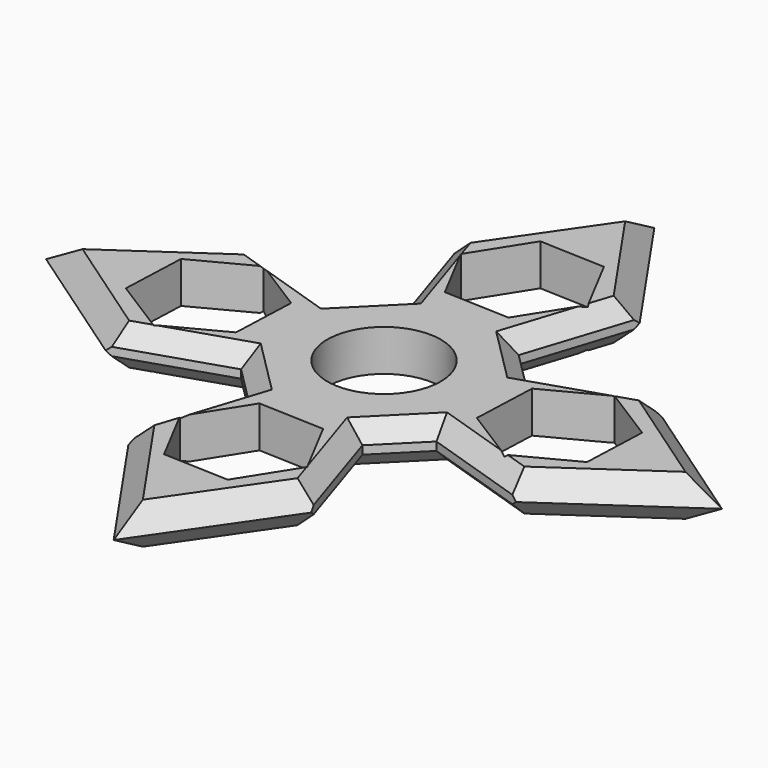
from build123d import *

# Parameters (mm, degrees)
F0_R          = 14.2875
F0_R_2        = 8.7122
F1_DEPTH      = 6.35
F2_T4_DEPTH   = 21.991422614
F2_T10_DEPTH  = 21.991422614
F2_T16_DEPTH  = 30.4110789775
F2_T21_DEPTH  = 30.4110789775
F2_T26_DEPTH  = 30.4110789775
F2_T31_DEPTH  = 30.4110789775
F2_T36_DEPTH  = 30.4110789775
F2_T41_DEPTH  = 30.4110789775
F2_T46_DEPTH  = 21.991422614
F2_T52_DEPTH  = 21.991422614
F2_T58_DEPTH  = 30.4110789775
F2_T63_DEPTH  = 30.4110789775
F2_T68_DEPTH  = 30.4110789775
F2_T73_DEPTH  = 30.4110789775
F2_T78_DEPTH  = 21.991422614
F2_T84_DEPTH  = 21.991422614
F2_T90_DEPTH  = 30.4110789775
F2_T95_DEPTH  = 30.4110789775
F2_T100_DEPTH = 30.4110789775
F2_T105_DEPTH = 30.4110789775
F2_T110_DEPTH = 21.991422614
F2_T116_DEPTH = 21.991422614
F2_T122_DEPTH = 30.4110789775
F2_T127_DEPTH = 30.4110789775
F2_T133_DEPTH = 30.4110789775
F2_T137_DEPTH = 21.991422614
F2_T144_DEPTH = 21.991422614
F2_T148_DEPTH = 30.4110789775
F2_T155_DEPTH = 30.4110789775
F2_T159_DEPTH = 21.991422614
F2_T166_DEPTH = 21.991422614
F2_T170_DEPTH = 30.4110789775
F2_T177_DEPTH = 30.4110789775
F2_T181_DEPTH = 21.991422614
F2_T188_DEPTH = 30.4110789775
F2_T192_DEPTH = 21.991422614
F2_T199_DEPTH = 21.991422614
F2_T203_DEPTH = 30.4110789775
F2_T210_DEPTH = 21.991422614
F2_T214_DEPTH = 30.4110789775
F2_T221_DEPTH = 30.4110789775
F2_T225_DEPTH = 21.991422614
F2_T232_DEPTH = 30.4110789775
F2_T236_DEPTH = 21.991422614
F2_T243_DEPTH = 21.991422614
F2_T247_DEPTH = 30.4110789775
F2_T254_DEPTH = 21.991422614
F2_T258_DEPTH = 30.4110789775
F2_T265_DEPTH = 30.4110789775
F2_T269_DEPTH = 21.991422614
F2_T276_DEPTH = 30.4110789775
F2_T280_DEPTH = 21.991422614
F2_T287_DEPTH = 21.991422614
F2_T291_DEPTH = 30.4110789775
F2_T298_DEPTH = 21.991422614
F2_T302_DEPTH = 30.4110789775
F3_SIZE       = 3.17499


# Not quite as in the source:
# - a fillet or chamfer that OpenCascade refuses, or shapes differently, is made with other operations: its cross-section is extruded or revolved along the edge and cut away or added
# - a fillet or chamfer is up to 0.001 mm smaller than in the source, because OpenCascade refuses the exact size


with BuildPart() as f1:
    # F0 (on Top) → F1 (new body)
    with BuildSketch(Plane.XY):
        Polygon((14.986, 8.6734646993), (8.6734646993, 14.986), (-8.6734646993, 14.986), (-14.986, 8.6734646993), (-14.986, -8.6734646993), (-8.6734646993, -14.986), (8.6734646993, -14.986), (14.986, -8.6734646993), align=None)
        Circle(F0_R, mode=Mode.SUBTRACT)
        Circle(F0_R)
        Circle(F0_R_2, mode=Mode.SUBTRACT)
        Polygon((-14.986, -8.6734646993), (-14.986, 8.6734646993), (-31.4839102423, 14.0339606837), (-41.6801795154, 0), (-31.4839102423, -14.0339606837), align=None)
        Polygon((-35.8485269353, -4.6903220641), (-35.4482015271, 5.3837060107), (-26.5236745918, 10.0740280748), (-17.9994730647, 4.6903220641), (-18.3997984729, -5.3837060107), (-27.3243254082, -10.0740280748), align=None, mode=Mode.SUBTRACT)
        Polygon((14.0339606837, -31.4839102423), (8.6734646993, -14.986), (-8.6734646993, -14.986), (-14.0339606837, -31.4839102423), (0, -41.6801795154), align=None)
        Polygon((4.6903220641, -35.8485269353), (-5.3837060107, -35.4482015271), (-10.0740280748, -26.5236745918), (-4.6903220641, -17.9994730647), (5.3837060107, -18.3997984729), (10.0740280748, -27.3243254082), align=None, mode=Mode.SUBTRACT)
        Polygon((31.4839102423, 14.0339606837), (14.986, 8.6734646993), (14.986, -8.6734646993), (31.4839102423, -14.0339606837), (41.6801795154, 0), align=None)
        Polygon((35.8485269353, 4.6903220641), (35.4482015271, -5.3837060107), (26.5236745918, -10.0740280748), (17.9994730647, -4.6903220641), (18.3997984729, 5.3837060107), (27.3243254082, 10.0740280748), align=None, mode=Mode.SUBTRACT)
        Polygon((-8.6734646993, 14.986), (8.6734646993, 14.986), (14.0339606837, 31.4839102423), (0, 41.6801795154), (-14.0339606837, 31.4839102423), align=None)
        Polygon((5.3837060107, 35.4482015271), (10.0740280748, 26.5236745918), (4.6903220641, 17.9994730647), (-5.3837060107, 18.3997984729), (-10.0740280748, 27.3243254082), (-4.6903220641, 35.8485269353), align=None, mode=Mode.SUBTRACT)
        Polygon((-41.6801795154, 0), (-31.4839102423, 14.0339606837), (-51.8401795154, 0), (-31.4839102423, -14.0339606837), align=None)
        Polygon((0, -51.8401795154), (14.0339606837, -31.4839102423), (0, -41.6801795154), (-14.0339606837, -31.4839102423), align=None)
        Polygon((51.8401795154, 0), (31.4839102423, 14.0339606837), (41.6801795154, 0), (31.4839102423, -14.0339606837), align=None)
        Polygon((0, 41.6801795154), (14.0339606837, 31.4839102423), (0, 51.8401795154), (-14.0339606837, 31.4839102423), align=None)
    extrude(amount=F1_DEPTH)

    # F2: chamfer of 2.54 on 24 edges, made by hand


with BuildPart() as f2_tool2:
    # F2_s3 → F2_t4 (new body)
    with BuildSketch(Plane(origin=(-7.7751420292, -7.7751420292, 0), x_dir=(0, 0, 1), z_dir=(0.7071067812, 0.7071067812, 0))):
        Polygon((3.81, 16.7297679281), (6.35, 14.1897679281), (6.35, 16.7297679281), align=None)
    extrude(amount=F2_T4_DEPTH)

    split(bisect_by=Plane(origin=(3.4409476252, 1.1180316571, 0), x_dir=(0, 0, 1), z_dir=(0.9510565163, 0.3090169944, 0)), keep=Keep.TOP)

    split(bisect_by=Plane(origin=(-1.1180316571, -3.4409476252, 0), x_dir=(0, 0, 1), z_dir=(-0.3090169944, -0.9510565163, 0)), keep=Keep.TOP)


with BuildPart() as f1_1:
    add(f1.part)

    # F2_t1: cut F2_tool2
    add(f2_tool2.part, mode=Mode.SUBTRACT)


with BuildPart() as f2_tool8:
    # F2_s9 → F2_t10 (new body)
    with BuildSketch(Plane(origin=(-7.7751420292, -7.7751420292, 0), x_dir=(0, 0, 1), z_dir=(0.7071067812, 0.7071067812, 0))):
        Polygon((2.54, 16.7297679281), (0, 14.1897679281), (0, 16.7297679281), align=None)
    extrude(amount=F2_T10_DEPTH)

    split(bisect_by=Plane(origin=(3.4409476252, 1.1180316571, 0), x_dir=(0, 0, 1), z_dir=(0.9510565163, 0.3090169944, 0)), keep=Keep.TOP)

    split(bisect_by=Plane(origin=(-1.1180316571, -3.4409476252, 0), x_dir=(0, 0, 1), z_dir=(-0.3090169944, -0.9510565163, 0)), keep=Keep.TOP)


with BuildPart() as f1_2:
    add(f1_1.part)

    # F2_t7: cut F2_tool8
    add(f2_tool8.part, mode=Mode.SUBTRACT)


with BuildPart() as f2_tool14:
    # F2_s15 → F2_t16 (new body)
    with BuildSketch(Plane(origin=(12.611535177, -38.8143141928, 0), x_dir=(0, 0, 1), z_dir=(-0.3090169944, 0.9510565163, 0))):
        Polygon((2.54, 3.6180264434), (0, 1.0780264434), (0, 3.6180264434), align=None)
    extrude(amount=F2_T16_DEPTH)

    split(bisect_by=Plane(origin=(11.8297323497, -11.8297323497, 0), x_dir=(0, 0, 1), z_dir=(0.7071067812, -0.7071067812, 0)), keep=Keep.TOP)


with BuildPart() as f1_3:
    add(f1_2.part)

    # F2_t13: cut F2_tool14
    add(f2_tool14.part, mode=Mode.SUBTRACT)


with BuildPart() as f2_tool19:
    # F2_s20 → F2_t21 (new body)
    with BuildSketch(Plane(origin=(12.611535177, -38.8143141928, 0), x_dir=(0, 0, 1), z_dir=(-0.3090169944, 0.9510565163, 0))):
        Polygon((3.81, 3.6180264434), (6.35, 1.0780264434), (6.35, 3.6180264434), align=None)
    extrude(amount=F2_T21_DEPTH)

    split(bisect_by=Plane(origin=(11.8297323497, -11.8297323497, 0), x_dir=(0, 0, 1), z_dir=(0.7071067812, -0.7071067812, 0)), keep=Keep.TOP)


with BuildPart() as f1_4:
    add(f1_3.part)

    # F2_t18: cut F2_tool19
    add(f2_tool19.part, mode=Mode.SUBTRACT)


with BuildPart() as f2_tool24:
    # F2_s25 → F2_t26 (new body)
    with BuildSketch(Plane(origin=(9.8916593637, -3.2139949557, 0), x_dir=(0, 0, 1), z_dir=(0.9510565163, -0.3090169944, 0))):
        Polygon((2.54, 3.6180264434), (0, 1.0780264434), (0, 3.6180264434), align=None)
    extrude(amount=F2_T26_DEPTH)

    split(bisect_by=Plane(origin=(11.8297323497, -11.8297323497, 0), x_dir=(0, 0, 1), z_dir=(0.7071067812, -0.7071067812, 0)), keep=Keep.TOP)


with BuildPart() as f1_5:
    add(f1_4.part)

    # F2_t23: cut F2_tool24
    add(f2_tool24.part, mode=Mode.SUBTRACT)


with BuildPart() as f2_tool29:
    # F2_s30 → F2_t31 (new body)
    with BuildSketch(Plane(origin=(9.8916593637, -3.2139949557, 0), x_dir=(0, 0, 1), z_dir=(0.9510565163, -0.3090169944, 0))):
        Polygon((3.81, 3.6180264434), (6.35, 1.0780264434), (6.35, 3.6180264434), align=None)
    extrude(amount=F2_T31_DEPTH)

    split(bisect_by=Plane(origin=(11.8297323497, -11.8297323497, 0), x_dir=(0, 0, 1), z_dir=(0.7071067812, -0.7071067812, 0)), keep=Keep.TOP)


with BuildPart() as f1_6:
    add(f1_5.part)

    # F2_t28: cut F2_tool29
    add(f2_tool29.part, mode=Mode.SUBTRACT)


with BuildPart() as f2_tool34:
    # F2_s35 → F2_t36 (new body)
    with BuildSketch(Plane(origin=(38.8143141928, 12.611535177, 0), x_dir=(0, 0, 1), z_dir=(-0.9510565163, -0.3090169944, 0))):
        Polygon((3.81, 3.6180264434), (6.35, 1.0780264434), (6.35, 3.6180264434), align=None)
    extrude(amount=F2_T36_DEPTH)

    split(bisect_by=Plane(origin=(11.8297323497, 11.8297323497, 0), x_dir=(0, 0, 1), z_dir=(0.7071067812, 0.7071067812, 0)), keep=Keep.TOP)


with BuildPart() as f1_7:
    add(f1_6.part)

    # F2_t33: cut F2_tool34
    add(f2_tool34.part, mode=Mode.SUBTRACT)


with BuildPart() as f2_tool39:
    # F2_s40 → F2_t41 (new body)
    with BuildSketch(Plane(origin=(38.8143141928, 12.611535177, 0), x_dir=(0, 0, 1), z_dir=(-0.9510565163, -0.3090169944, 0))):
        Polygon((2.54, 3.6180264434), (0, 1.0780264434), (0, 3.6180264434), align=None)
    extrude(amount=F2_T41_DEPTH)

    split(bisect_by=Plane(origin=(11.8297323497, 11.8297323497, 0), x_dir=(0, 0, 1), z_dir=(0.7071067812, 0.7071067812, 0)), keep=Keep.TOP)


with BuildPart() as f1_8:
    add(f1_7.part)

    # F2_t38: cut F2_tool39
    add(f2_tool39.part, mode=Mode.SUBTRACT)


with BuildPart() as f2_tool44:
    # F2_s45 → F2_t46 (new body)
    with BuildSketch(Plane(origin=(7.7751420292, -7.7751420292, 0), x_dir=(0, 0, 1), z_dir=(-0.7071067812, 0.7071067812, 0))):
        Polygon((2.54, 16.7297679281), (0, 14.1897679281), (0, 16.7297679281), align=None)
    extrude(amount=F2_T46_DEPTH)

    split(bisect_by=Plane(origin=(-1.1180316571, 3.4409476252, 0), x_dir=(0, 0, 1), z_dir=(-0.3090169944, 0.9510565163, 0)), keep=Keep.TOP)

    split(bisect_by=Plane(origin=(3.4409476252, -1.1180316571, 0), x_dir=(0, 0, 1), z_dir=(0.9510565163, -0.3090169944, 0)), keep=Keep.TOP)


with BuildPart() as f1_9:
    add(f1_8.part)

    # F2_t43: cut F2_tool44
    add(f2_tool44.part, mode=Mode.SUBTRACT)


with BuildPart() as f2_tool50:
    # F2_s51 → F2_t52 (new body)
    with BuildSketch(Plane(origin=(7.7751420292, -7.7751420292, 0), x_dir=(0, 0, 1), z_dir=(-0.7071067812, 0.7071067812, 0))):
        Polygon((3.81, 16.7297679281), (6.35, 14.1897679281), (6.35, 16.7297679281), align=None)
    extrude(amount=F2_T52_DEPTH)

    split(bisect_by=Plane(origin=(-1.1180316571, 3.4409476252, 0), x_dir=(0, 0, 1), z_dir=(-0.3090169944, 0.9510565163, 0)), keep=Keep.TOP)

    split(bisect_by=Plane(origin=(3.4409476252, -1.1180316571, 0), x_dir=(0, 0, 1), z_dir=(0.9510565163, -0.3090169944, 0)), keep=Keep.TOP)


with BuildPart() as f1_10:
    add(f1_9.part)

    # F2_t49: cut F2_tool50
    add(f2_tool50.part, mode=Mode.SUBTRACT)


with BuildPart() as f2_tool56:
    # F2_s57 → F2_t58 (new body)
    with BuildSketch(Plane(origin=(3.2139949557, 9.8916593637, 0), x_dir=(0, 0, 1), z_dir=(0.3090169944, 0.9510565163, 0))):
        Polygon((2.54, 3.6180264434), (0, 1.0780264434), (0, 3.6180264434), align=None)
    extrude(amount=F2_T58_DEPTH)

    split(bisect_by=Plane(origin=(11.8297323497, 11.8297323497, 0), x_dir=(0, 0, 1), z_dir=(0.7071067812, 0.7071067812, 0)), keep=Keep.TOP)


with BuildPart() as f1_11:
    add(f1_10.part)

    # F2_t55: cut F2_tool56
    add(f2_tool56.part, mode=Mode.SUBTRACT)


with BuildPart() as f2_tool61:
    # F2_s62 → F2_t63 (new body)
    with BuildSketch(Plane(origin=(3.2139949557, 9.8916593637, 0), x_dir=(0, 0, 1), z_dir=(0.3090169944, 0.9510565163, 0))):
        Polygon((3.81, 3.6180264434), (6.35, 1.0780264434), (6.35, 3.6180264434), align=None)
    extrude(amount=F2_T63_DEPTH)

    split(bisect_by=Plane(origin=(11.8297323497, 11.8297323497, 0), x_dir=(0, 0, 1), z_dir=(0.7071067812, 0.7071067812, 0)), keep=Keep.TOP)


with BuildPart() as f1_12:
    add(f1_11.part)

    # F2_t60: cut F2_tool61
    add(f2_tool61.part, mode=Mode.SUBTRACT)


with BuildPart() as f2_tool66:
    # F2_s67 → F2_t68 (new body)
    with BuildSketch(Plane(origin=(-12.611535177, 38.8143141928, 0), x_dir=(0, 0, 1), z_dir=(0.3090169944, -0.9510565163, 0))):
        Polygon((3.81, 3.6180264434), (6.35, 1.0780264434), (6.35, 3.6180264434), align=None)
    extrude(amount=F2_T68_DEPTH)

    split(bisect_by=Plane(origin=(-11.8297323497, 11.8297323497, 0), x_dir=(0, 0, 1), z_dir=(-0.7071067812, 0.7071067812, 0)), keep=Keep.TOP)


with BuildPart() as f1_13:
    add(f1_12.part)

    # F2_t65: cut F2_tool66
    add(f2_tool66.part, mode=Mode.SUBTRACT)


with BuildPart() as f2_tool71:
    # F2_s72 → F2_t73 (new body)
    with BuildSketch(Plane(origin=(-12.611535177, 38.8143141928, 0), x_dir=(0, 0, 1), z_dir=(0.3090169944, -0.9510565163, 0))):
        Polygon((2.54, 3.6180264434), (0, 1.0780264434), (0, 3.6180264434), align=None)
    extrude(amount=F2_T73_DEPTH)

    split(bisect_by=Plane(origin=(-11.8297323497, 11.8297323497, 0), x_dir=(0, 0, 1), z_dir=(-0.7071067812, 0.7071067812, 0)), keep=Keep.TOP)


with BuildPart() as f1_14:
    add(f1_13.part)

    # F2_t70: cut F2_tool71
    add(f2_tool71.part, mode=Mode.SUBTRACT)


with BuildPart() as f2_tool76:
    # F2_s77 → F2_t78 (new body)
    with BuildSketch(Plane(origin=(7.7751420292, 7.7751420292, 0), x_dir=(0, 0, 1), z_dir=(-0.7071067812, -0.7071067812, 0))):
        Polygon((3.81, 16.7297679281), (6.35, 14.1897679281), (6.35, 16.7297679281), align=None)
    extrude(amount=F2_T78_DEPTH)

    split(bisect_by=Plane(origin=(-3.4409476252, -1.1180316571, 0), x_dir=(0, 0, 1), z_dir=(-0.9510565163, -0.3090169944, 0)), keep=Keep.TOP)

    split(bisect_by=Plane(origin=(1.1180316571, 3.4409476252, 0), x_dir=(0, 0, 1), z_dir=(0.3090169944, 0.9510565163, 0)), keep=Keep.TOP)


with BuildPart() as f1_15:
    add(f1_14.part)

    # F2_t75: cut F2_tool76
    add(f2_tool76.part, mode=Mode.SUBTRACT)


with BuildPart() as f2_tool82:
    # F2_s83 → F2_t84 (new body)
    with BuildSketch(Plane(origin=(7.7751420292, 7.7751420292, 0), x_dir=(0, 0, 1), z_dir=(-0.7071067812, -0.7071067812, 0))):
        Polygon((2.54, 16.7297679281), (0, 14.1897679281), (0, 16.7297679281), align=None)
    extrude(amount=F2_T84_DEPTH)

    split(bisect_by=Plane(origin=(-3.4409476252, -1.1180316571, 0), x_dir=(0, 0, 1), z_dir=(-0.9510565163, -0.3090169944, 0)), keep=Keep.TOP)

    split(bisect_by=Plane(origin=(1.1180316571, 3.4409476252, 0), x_dir=(0, 0, 1), z_dir=(0.3090169944, 0.9510565163, 0)), keep=Keep.TOP)


with BuildPart() as f1_16:
    add(f1_15.part)

    # F2_t81: cut F2_tool82
    add(f2_tool82.part, mode=Mode.SUBTRACT)


with BuildPart() as f2_tool88:
    # F2_s89 → F2_t90 (new body)
    with BuildSketch(Plane(origin=(-9.8916593637, 3.2139949557, 0), x_dir=(0, 0, 1), z_dir=(-0.9510565163, 0.3090169944, 0))):
        Polygon((2.54, 3.6180264434), (0, 1.0780264434), (0, 3.6180264434), align=None)
    extrude(amount=F2_T90_DEPTH)

    split(bisect_by=Plane(origin=(-11.8297323497, 11.8297323497, 0), x_dir=(0, 0, 1), z_dir=(-0.7071067812, 0.7071067812, 0)), keep=Keep.TOP)


with BuildPart() as f1_17:
    add(f1_16.part)

    # F2_t87: cut F2_tool88
    add(f2_tool88.part, mode=Mode.SUBTRACT)


with BuildPart() as f2_tool93:
    # F2_s94 → F2_t95 (new body)
    with BuildSketch(Plane(origin=(-9.8916593637, 3.2139949557, 0), x_dir=(0, 0, 1), z_dir=(-0.9510565163, 0.3090169944, 0))):
        Polygon((3.81, 3.6180264434), (6.35, 1.0780264434), (6.35, 3.6180264434), align=None)
    extrude(amount=F2_T95_DEPTH)

    split(bisect_by=Plane(origin=(-11.8297323497, 11.8297323497, 0), x_dir=(0, 0, 1), z_dir=(-0.7071067812, 0.7071067812, 0)), keep=Keep.TOP)


with BuildPart() as f1_18:
    add(f1_17.part)

    # F2_t92: cut F2_tool93
    add(f2_tool93.part, mode=Mode.SUBTRACT)


with BuildPart() as f2_tool98:
    # F2_s99 → F2_t100 (new body)
    with BuildSketch(Plane(origin=(-38.8143141928, -12.611535177, 0), x_dir=(0, 0, 1), z_dir=(0.9510565163, 0.3090169944, 0))):
        Polygon((3.81, 3.6180264434), (6.35, 1.0780264434), (6.35, 3.6180264434), align=None)
    extrude(amount=F2_T100_DEPTH)

    split(bisect_by=Plane(origin=(-11.8297323497, -11.8297323497, 0), x_dir=(0, 0, 1), z_dir=(-0.7071067812, -0.7071067812, 0)), keep=Keep.TOP)


with BuildPart() as f1_19:
    add(f1_18.part)

    # F2_t97: cut F2_tool98
    add(f2_tool98.part, mode=Mode.SUBTRACT)


with BuildPart() as f2_tool103:
    # F2_s104 → F2_t105 (new body)
    with BuildSketch(Plane(origin=(-38.8143141928, -12.611535177, 0), x_dir=(0, 0, 1), z_dir=(0.9510565163, 0.3090169944, 0))):
        Polygon((2.54, 3.6180264434), (0, 1.0780264434), (0, 3.6180264434), align=None)
    extrude(amount=F2_T105_DEPTH)

    split(bisect_by=Plane(origin=(-11.8297323497, -11.8297323497, 0), x_dir=(0, 0, 1), z_dir=(-0.7071067812, -0.7071067812, 0)), keep=Keep.TOP)


with BuildPart() as f1_20:
    add(f1_19.part)

    # F2_t102: cut F2_tool103
    add(f2_tool103.part, mode=Mode.SUBTRACT)


with BuildPart() as f2_tool108:
    # F2_s109 → F2_t110 (new body)
    with BuildSketch(Plane(origin=(-7.7751420292, 7.7751420292, 0), x_dir=(0, 0, 1), z_dir=(0.7071067812, -0.7071067812, 0))):
        Polygon((3.81, 16.7297679281), (6.35, 14.1897679281), (6.35, 16.7297679281), align=None)
    extrude(amount=F2_T110_DEPTH)

    split(bisect_by=Plane(origin=(1.1180316571, -3.4409476252, 0), x_dir=(0, 0, 1), z_dir=(0.3090169944, -0.9510565163, 0)), keep=Keep.TOP)

    split(bisect_by=Plane(origin=(-3.4409476252, 1.1180316571, 0), x_dir=(0, 0, 1), z_dir=(-0.9510565163, 0.3090169944, 0)), keep=Keep.TOP)


with BuildPart() as f1_21:
    add(f1_20.part)

    # F2_t107: cut F2_tool108
    add(f2_tool108.part, mode=Mode.SUBTRACT)


with BuildPart() as f2_tool114:
    # F2_s115 → F2_t116 (new body)
    with BuildSketch(Plane(origin=(-7.7751420292, 7.7751420292, 0), x_dir=(0, 0, 1), z_dir=(0.7071067812, -0.7071067812, 0))):
        Polygon((2.54, 16.7297679281), (0, 14.1897679281), (0, 16.7297679281), align=None)
    extrude(amount=F2_T116_DEPTH)

    split(bisect_by=Plane(origin=(1.1180316571, -3.4409476252, 0), x_dir=(0, 0, 1), z_dir=(0.3090169944, -0.9510565163, 0)), keep=Keep.TOP)

    split(bisect_by=Plane(origin=(-3.4409476252, 1.1180316571, 0), x_dir=(0, 0, 1), z_dir=(-0.9510565163, 0.3090169944, 0)), keep=Keep.TOP)


with BuildPart() as f1_22:
    add(f1_21.part)

    # F2_t113: cut F2_tool114
    add(f2_tool114.part, mode=Mode.SUBTRACT)


with BuildPart() as f2_tool120:
    # F2_s121 → F2_t122 (new body)
    with BuildSketch(Plane(origin=(-3.2139949557, -9.8916593637, 0), x_dir=(0, 0, 1), z_dir=(-0.3090169944, -0.9510565163, 0))):
        Polygon((3.81, 3.6180264434), (6.35, 1.0780264434), (6.35, 3.6180264434), align=None)
    extrude(amount=F2_T122_DEPTH)

    split(bisect_by=Plane(origin=(-11.8297323497, -11.8297323497, 0), x_dir=(0, 0, 1), z_dir=(-0.7071067812, -0.7071067812, 0)), keep=Keep.TOP)


with BuildPart() as f1_23:
    add(f1_22.part)

    # F2_t119: cut F2_tool120
    add(f2_tool120.part, mode=Mode.SUBTRACT)


with BuildPart() as f2_tool125:
    # F2_s126 → F2_t127 (new body)
    with BuildSketch(Plane(origin=(-3.2139949557, -9.8916593637, 0), x_dir=(0, 0, 1), z_dir=(-0.3090169944, -0.9510565163, 0))):
        Polygon((2.54, 3.6180264434), (0, 1.0780264434), (0, 3.6180264434), align=None)
    extrude(amount=F2_T127_DEPTH)

    split(bisect_by=Plane(origin=(-11.8297323497, -11.8297323497, 0), x_dir=(0, 0, 1), z_dir=(-0.7071067812, -0.7071067812, 0)), keep=Keep.TOP)


with BuildPart() as f1_24:
    add(f1_23.part)

    # F2_t124: cut F2_tool125
    add(f2_tool125.part, mode=Mode.SUBTRACT)


with BuildPart() as f2_tool131:
    # F2_s132 → F2_t133 (new body)
    with BuildSketch(Plane(origin=(12.611535177, -38.8143141928, 0), x_dir=(0, 0, 1), z_dir=(-0.3090169944, 0.9510565163, 0))):
        Polygon((3.81, 3.6180264434), (6.35, 1.0780264434), (6.35, 3.6180264434), align=None)
    extrude(amount=F2_T133_DEPTH)

    split(bisect_by=Plane(origin=(11.8297323497, -11.8297323497, 0), x_dir=(0, 0, 1), z_dir=(-0.7071067812, 0.7071067812, 0)), keep=Keep.TOP)


with BuildPart() as f2_tool135:
    # F2_s136 → F2_t137 (new body)
    with BuildSketch(Plane(origin=(-7.7751420292, -7.7751420292, 0), x_dir=(0, 0, 1), z_dir=(0.7071067812, 0.7071067812, 0))):
        Polygon((3.81, 16.7297679281), (6.35, 14.1897679281), (6.35, 16.7297679281), align=None)
    extrude(amount=F2_T137_DEPTH)

    split(bisect_by=Plane(origin=(3.4409476252, 1.1180316571, 0), x_dir=(0, 0, 1), z_dir=(-0.9510565163, -0.3090169944, 0)), keep=Keep.TOP)


with BuildPart() as f2_tool131_1:
    add(f2_tool131.part)

    # F2_t139: intersect F2_tool135
    add(f2_tool135.part, mode=Mode.INTERSECT)


with BuildPart() as f1_25:
    add(f1_24.part)

    # F2_t129: cut F2_tool131
    add(f2_tool131_1.part, mode=Mode.SUBTRACT)


with BuildPart() as f2_tool142:
    # F2_s143 → F2_t144 (new body)
    with BuildSketch(Plane(origin=(-7.7751420292, -7.7751420292, 0), x_dir=(0, 0, 1), z_dir=(0.7071067812, 0.7071067812, 0))):
        Polygon((3.81, 16.7297679281), (6.35, 14.1897679281), (6.35, 16.7297679281), align=None)
    extrude(amount=F2_T144_DEPTH)

    split(bisect_by=Plane(origin=(-1.1180316571, -3.4409476252, 0), x_dir=(0, 0, 1), z_dir=(0.3090169944, 0.9510565163, 0)), keep=Keep.TOP)


with BuildPart() as f2_tool146:
    # F2_s147 → F2_t148 (new body)
    with BuildSketch(Plane(origin=(9.8916593637, -3.2139949557, 0), x_dir=(0, 0, 1), z_dir=(0.9510565163, -0.3090169944, 0))):
        Polygon((3.81, 3.6180264434), (6.35, 1.0780264434), (6.35, 3.6180264434), align=None)
    extrude(amount=F2_T148_DEPTH)

    split(bisect_by=Plane(origin=(11.8297323497, -11.8297323497, 0), x_dir=(0, 0, 1), z_dir=(-0.7071067812, 0.7071067812, 0)), keep=Keep.TOP)


with BuildPart() as f2_tool142_1:
    add(f2_tool142.part)

    # F2_t150: intersect F2_tool146
    add(f2_tool146.part, mode=Mode.INTERSECT)


with BuildPart() as f1_26:
    add(f1_25.part)

    # F2_t140: cut F2_tool142
    add(f2_tool142_1.part, mode=Mode.SUBTRACT)


with BuildPart() as f2_tool153:
    # F2_s154 → F2_t155 (new body)
    with BuildSketch(Plane(origin=(12.611535177, -38.8143141928, 0), x_dir=(0, 0, 1), z_dir=(-0.3090169944, 0.9510565163, 0))):
        Polygon((2.54, 3.6180264434), (0, 1.0780264434), (0, 3.6180264434), align=None)
    extrude(amount=F2_T155_DEPTH)

    split(bisect_by=Plane(origin=(11.8297323497, -11.8297323497, 0), x_dir=(0, 0, 1), z_dir=(-0.7071067812, 0.7071067812, 0)), keep=Keep.TOP)


with BuildPart() as f2_tool157:
    # F2_s158 → F2_t159 (new body)
    with BuildSketch(Plane(origin=(-7.7751420292, -7.7751420292, 0), x_dir=(0, 0, 1), z_dir=(0.7071067812, 0.7071067812, 0))):
        Polygon((2.54, 16.7297679281), (0, 14.1897679281), (0, 16.7297679281), align=None)
    extrude(amount=F2_T159_DEPTH)

    split(bisect_by=Plane(origin=(3.4409476252, 1.1180316571, 0), x_dir=(0, 0, 1), z_dir=(-0.9510565163, -0.3090169944, 0)), keep=Keep.TOP)


with BuildPart() as f2_tool153_1:
    add(f2_tool153.part)

    # F2_t161: intersect F2_tool157
    add(f2_tool157.part, mode=Mode.INTERSECT)


with BuildPart() as f1_27:
    add(f1_26.part)

    # F2_t151: cut F2_tool153
    add(f2_tool153_1.part, mode=Mode.SUBTRACT)


with BuildPart() as f2_tool164:
    # F2_s165 → F2_t166 (new body)
    with BuildSketch(Plane(origin=(-7.7751420292, -7.7751420292, 0), x_dir=(0, 0, 1), z_dir=(0.7071067812, 0.7071067812, 0))):
        Polygon((2.54, 16.7297679281), (0, 14.1897679281), (0, 16.7297679281), align=None)
    extrude(amount=F2_T166_DEPTH)

    split(bisect_by=Plane(origin=(-1.1180316571, -3.4409476252, 0), x_dir=(0, 0, 1), z_dir=(0.3090169944, 0.9510565163, 0)), keep=Keep.TOP)


with BuildPart() as f2_tool168:
    # F2_s169 → F2_t170 (new body)
    with BuildSketch(Plane(origin=(9.8916593637, -3.2139949557, 0), x_dir=(0, 0, 1), z_dir=(0.9510565163, -0.3090169944, 0))):
        Polygon((2.54, 3.6180264434), (0, 1.0780264434), (0, 3.6180264434), align=None)
    extrude(amount=F2_T170_DEPTH)

    split(bisect_by=Plane(origin=(11.8297323497, -11.8297323497, 0), x_dir=(0, 0, 1), z_dir=(-0.7071067812, 0.7071067812, 0)), keep=Keep.TOP)


with BuildPart() as f2_tool164_1:
    add(f2_tool164.part)

    # F2_t172: intersect F2_tool168
    add(f2_tool168.part, mode=Mode.INTERSECT)


with BuildPart() as f1_28:
    add(f1_27.part)

    # F2_t162: cut F2_tool164
    add(f2_tool164_1.part, mode=Mode.SUBTRACT)


with BuildPart() as f2_tool175:
    # F2_s176 → F2_t177 (new body)
    with BuildSketch(Plane(origin=(38.8143141928, 12.611535177, 0), x_dir=(0, 0, 1), z_dir=(-0.9510565163, -0.3090169944, 0))):
        Polygon((3.81, 3.6180264434), (6.35, 1.0780264434), (6.35, 3.6180264434), align=None)
    extrude(amount=F2_T177_DEPTH)

    split(bisect_by=Plane(origin=(11.8297323497, 11.8297323497, 0), x_dir=(0, 0, 1), z_dir=(-0.7071067812, -0.7071067812, 0)), keep=Keep.TOP)


with BuildPart() as f2_tool179:
    # F2_s180 → F2_t181 (new body)
    with BuildSketch(Plane(origin=(7.7751420292, -7.7751420292, 0), x_dir=(0, 0, 1), z_dir=(-0.7071067812, 0.7071067812, 0))):
        Polygon((3.81, 16.7297679281), (6.35, 14.1897679281), (6.35, 16.7297679281), align=None)
    extrude(amount=F2_T181_DEPTH)

    split(bisect_by=Plane(origin=(-1.1180316571, 3.4409476252, 0), x_dir=(0, 0, 1), z_dir=(0.3090169944, -0.9510565163, 0)), keep=Keep.TOP)


with BuildPart() as f2_tool175_1:
    add(f2_tool175.part)

    # F2_t183: intersect F2_tool179
    add(f2_tool179.part, mode=Mode.INTERSECT)


with BuildPart() as f1_29:
    add(f1_28.part)

    # F2_t173: cut F2_tool175
    add(f2_tool175_1.part, mode=Mode.SUBTRACT)


with BuildPart() as f2_tool186:
    # F2_s187 → F2_t188 (new body)
    with BuildSketch(Plane(origin=(38.8143141928, 12.611535177, 0), x_dir=(0, 0, 1), z_dir=(-0.9510565163, -0.3090169944, 0))):
        Polygon((2.54, 3.6180264434), (0, 1.0780264434), (0, 3.6180264434), align=None)
    extrude(amount=F2_T188_DEPTH)

    split(bisect_by=Plane(origin=(11.8297323497, 11.8297323497, 0), x_dir=(0, 0, 1), z_dir=(-0.7071067812, -0.7071067812, 0)), keep=Keep.TOP)


with BuildPart() as f2_tool190:
    # F2_s191 → F2_t192 (new body)
    with BuildSketch(Plane(origin=(7.7751420292, -7.7751420292, 0), x_dir=(0, 0, 1), z_dir=(-0.7071067812, 0.7071067812, 0))):
        Polygon((2.54, 16.7297679281), (0, 14.1897679281), (0, 16.7297679281), align=None)
    extrude(amount=F2_T192_DEPTH)

    split(bisect_by=Plane(origin=(-1.1180316571, 3.4409476252, 0), x_dir=(0, 0, 1), z_dir=(0.3090169944, -0.9510565163, 0)), keep=Keep.TOP)


with BuildPart() as f2_tool186_1:
    add(f2_tool186.part)

    # F2_t194: intersect F2_tool190
    add(f2_tool190.part, mode=Mode.INTERSECT)


with BuildPart() as f1_30:
    add(f1_29.part)

    # F2_t184: cut F2_tool186
    add(f2_tool186_1.part, mode=Mode.SUBTRACT)


with BuildPart() as f2_tool197:
    # F2_s198 → F2_t199 (new body)
    with BuildSketch(Plane(origin=(7.7751420292, -7.7751420292, 0), x_dir=(0, 0, 1), z_dir=(-0.7071067812, 0.7071067812, 0))):
        Polygon((2.54, 16.7297679281), (0, 14.1897679281), (0, 16.7297679281), align=None)
    extrude(amount=F2_T199_DEPTH)

    split(bisect_by=Plane(origin=(3.4409476252, -1.1180316571, 0), x_dir=(0, 0, 1), z_dir=(-0.9510565163, 0.3090169944, 0)), keep=Keep.TOP)


with BuildPart() as f2_tool201:
    # F2_s202 → F2_t203 (new body)
    with BuildSketch(Plane(origin=(3.2139949557, 9.8916593637, 0), x_dir=(0, 0, 1), z_dir=(0.3090169944, 0.9510565163, 0))):
        Polygon((2.54, 3.6180264434), (0, 1.0780264434), (0, 3.6180264434), align=None)
    extrude(amount=F2_T203_DEPTH)

    split(bisect_by=Plane(origin=(11.8297323497, 11.8297323497, 0), x_dir=(0, 0, 1), z_dir=(-0.7071067812, -0.7071067812, 0)), keep=Keep.TOP)


with BuildPart() as f2_tool197_1:
    add(f2_tool197.part)

    # F2_t205: intersect F2_tool201
    add(f2_tool201.part, mode=Mode.INTERSECT)


with BuildPart() as f1_31:
    add(f1_30.part)

    # F2_t195: cut F2_tool197
    add(f2_tool197_1.part, mode=Mode.SUBTRACT)


with BuildPart() as f2_tool208:
    # F2_s209 → F2_t210 (new body)
    with BuildSketch(Plane(origin=(7.7751420292, -7.7751420292, 0), x_dir=(0, 0, 1), z_dir=(-0.7071067812, 0.7071067812, 0))):
        Polygon((3.81, 16.7297679281), (6.35, 14.1897679281), (6.35, 16.7297679281), align=None)
    extrude(amount=F2_T210_DEPTH)

    split(bisect_by=Plane(origin=(3.4409476252, -1.1180316571, 0), x_dir=(0, 0, 1), z_dir=(-0.9510565163, 0.3090169944, 0)), keep=Keep.TOP)


with BuildPart() as f2_tool212:
    # F2_s213 → F2_t214 (new body)
    with BuildSketch(Plane(origin=(3.2139949557, 9.8916593637, 0), x_dir=(0, 0, 1), z_dir=(0.3090169944, 0.9510565163, 0))):
        Polygon((3.81, 3.6180264434), (6.35, 1.0780264434), (6.35, 3.6180264434), align=None)
    extrude(amount=F2_T214_DEPTH)

    split(bisect_by=Plane(origin=(11.8297323497, 11.8297323497, 0), x_dir=(0, 0, 1), z_dir=(-0.7071067812, -0.7071067812, 0)), keep=Keep.TOP)


with BuildPart() as f2_tool208_1:
    add(f2_tool208.part)

    # F2_t216: intersect F2_tool212
    add(f2_tool212.part, mode=Mode.INTERSECT)


with BuildPart() as f1_32:
    add(f1_31.part)

    # F2_t206: cut F2_tool208
    add(f2_tool208_1.part, mode=Mode.SUBTRACT)


with BuildPart() as f2_tool219:
    # F2_s220 → F2_t221 (new body)
    with BuildSketch(Plane(origin=(-12.611535177, 38.8143141928, 0), x_dir=(0, 0, 1), z_dir=(0.3090169944, -0.9510565163, 0))):
        Polygon((3.81, 3.6180264434), (6.35, 1.0780264434), (6.35, 3.6180264434), align=None)
    extrude(amount=F2_T221_DEPTH)

    split(bisect_by=Plane(origin=(-11.8297323497, 11.8297323497, 0), x_dir=(0, 0, 1), z_dir=(0.7071067812, -0.7071067812, 0)), keep=Keep.TOP)


with BuildPart() as f2_tool223:
    # F2_s224 → F2_t225 (new body)
    with BuildSketch(Plane(origin=(7.7751420292, 7.7751420292, 0), x_dir=(0, 0, 1), z_dir=(-0.7071067812, -0.7071067812, 0))):
        Polygon((3.81, 16.7297679281), (6.35, 14.1897679281), (6.35, 16.7297679281), align=None)
    extrude(amount=F2_T225_DEPTH)

    split(bisect_by=Plane(origin=(-3.4409476252, -1.1180316571, 0), x_dir=(0, 0, 1), z_dir=(0.9510565163, 0.3090169944, 0)), keep=Keep.TOP)


with BuildPart() as f2_tool219_1:
    add(f2_tool219.part)

    # F2_t227: intersect F2_tool223
    add(f2_tool223.part, mode=Mode.INTERSECT)


with BuildPart() as f1_33:
    add(f1_32.part)

    # F2_t217: cut F2_tool219
    add(f2_tool219_1.part, mode=Mode.SUBTRACT)


with BuildPart() as f2_tool230:
    # F2_s231 → F2_t232 (new body)
    with BuildSketch(Plane(origin=(-12.611535177, 38.8143141928, 0), x_dir=(0, 0, 1), z_dir=(0.3090169944, -0.9510565163, 0))):
        Polygon((2.54, 3.6180264434), (0, 1.0780264434), (0, 3.6180264434), align=None)
    extrude(amount=F2_T232_DEPTH)

    split(bisect_by=Plane(origin=(-11.8297323497, 11.8297323497, 0), x_dir=(0, 0, 1), z_dir=(0.7071067812, -0.7071067812, 0)), keep=Keep.TOP)


with BuildPart() as f2_tool234:
    # F2_s235 → F2_t236 (new body)
    with BuildSketch(Plane(origin=(7.7751420292, 7.7751420292, 0), x_dir=(0, 0, 1), z_dir=(-0.7071067812, -0.7071067812, 0))):
        Polygon((2.54, 16.7297679281), (0, 14.1897679281), (0, 16.7297679281), align=None)
    extrude(amount=F2_T236_DEPTH)

    split(bisect_by=Plane(origin=(-3.4409476252, -1.1180316571, 0), x_dir=(0, 0, 1), z_dir=(0.9510565163, 0.3090169944, 0)), keep=Keep.TOP)


with BuildPart() as f2_tool230_1:
    add(f2_tool230.part)

    # F2_t238: intersect F2_tool234
    add(f2_tool234.part, mode=Mode.INTERSECT)


with BuildPart() as f1_34:
    add(f1_33.part)

    # F2_t228: cut F2_tool230
    add(f2_tool230_1.part, mode=Mode.SUBTRACT)


with BuildPart() as f2_tool241:
    # F2_s242 → F2_t243 (new body)
    with BuildSketch(Plane(origin=(7.7751420292, 7.7751420292, 0), x_dir=(0, 0, 1), z_dir=(-0.7071067812, -0.7071067812, 0))):
        Polygon((3.81, 16.7297679281), (6.35, 14.1897679281), (6.35, 16.7297679281), align=None)
    extrude(amount=F2_T243_DEPTH)

    split(bisect_by=Plane(origin=(1.1180316571, 3.4409476252, 0), x_dir=(0, 0, 1), z_dir=(-0.3090169944, -0.9510565163, 0)), keep=Keep.TOP)


with BuildPart() as f2_tool245:
    # F2_s246 → F2_t247 (new body)
    with BuildSketch(Plane(origin=(-9.8916593637, 3.2139949557, 0), x_dir=(0, 0, 1), z_dir=(-0.9510565163, 0.3090169944, 0))):
        Polygon((3.81, 3.6180264434), (6.35, 1.0780264434), (6.35, 3.6180264434), align=None)
    extrude(amount=F2_T247_DEPTH)

    split(bisect_by=Plane(origin=(-11.8297323497, 11.8297323497, 0), x_dir=(0, 0, 1), z_dir=(0.7071067812, -0.7071067812, 0)), keep=Keep.TOP)


with BuildPart() as f2_tool241_1:
    add(f2_tool241.part)

    # F2_t249: intersect F2_tool245
    add(f2_tool245.part, mode=Mode.INTERSECT)


with BuildPart() as f1_35:
    add(f1_34.part)

    # F2_t239: cut F2_tool241
    add(f2_tool241_1.part, mode=Mode.SUBTRACT)


with BuildPart() as f2_tool252:
    # F2_s253 → F2_t254 (new body)
    with BuildSketch(Plane(origin=(7.7751420292, 7.7751420292, 0), x_dir=(0, 0, 1), z_dir=(-0.7071067812, -0.7071067812, 0))):
        Polygon((2.54, 16.7297679281), (0, 14.1897679281), (0, 16.7297679281), align=None)
    extrude(amount=F2_T254_DEPTH)

    split(bisect_by=Plane(origin=(1.1180316571, 3.4409476252, 0), x_dir=(0, 0, 1), z_dir=(-0.3090169944, -0.9510565163, 0)), keep=Keep.TOP)


with BuildPart() as f2_tool256:
    # F2_s257 → F2_t258 (new body)
    with BuildSketch(Plane(origin=(-9.8916593637, 3.2139949557, 0), x_dir=(0, 0, 1), z_dir=(-0.9510565163, 0.3090169944, 0))):
        Polygon((2.54, 3.6180264434), (0, 1.0780264434), (0, 3.6180264434), align=None)
    extrude(amount=F2_T258_DEPTH)

    split(bisect_by=Plane(origin=(-11.8297323497, 11.8297323497, 0), x_dir=(0, 0, 1), z_dir=(0.7071067812, -0.7071067812, 0)), keep=Keep.TOP)


with BuildPart() as f2_tool252_1:
    add(f2_tool252.part)

    # F2_t260: intersect F2_tool256
    add(f2_tool256.part, mode=Mode.INTERSECT)


with BuildPart() as f1_36:
    add(f1_35.part)

    # F2_t250: cut F2_tool252
    add(f2_tool252_1.part, mode=Mode.SUBTRACT)


with BuildPart() as f2_tool263:
    # F2_s264 → F2_t265 (new body)
    with BuildSketch(Plane(origin=(-38.8143141928, -12.611535177, 0), x_dir=(0, 0, 1), z_dir=(0.9510565163, 0.3090169944, 0))):
        Polygon((3.81, 3.6180264434), (6.35, 1.0780264434), (6.35, 3.6180264434), align=None)
    extrude(amount=F2_T265_DEPTH)

    split(bisect_by=Plane(origin=(-11.8297323497, -11.8297323497, 0), x_dir=(0, 0, 1), z_dir=(0.7071067812, 0.7071067812, 0)), keep=Keep.TOP)


with BuildPart() as f2_tool267:
    # F2_s268 → F2_t269 (new body)
    with BuildSketch(Plane(origin=(-7.7751420292, 7.7751420292, 0), x_dir=(0, 0, 1), z_dir=(0.7071067812, -0.7071067812, 0))):
        Polygon((3.81, 16.7297679281), (6.35, 14.1897679281), (6.35, 16.7297679281), align=None)
    extrude(amount=F2_T269_DEPTH)

    split(bisect_by=Plane(origin=(1.1180316571, -3.4409476252, 0), x_dir=(0, 0, 1), z_dir=(-0.3090169944, 0.9510565163, 0)), keep=Keep.TOP)


with BuildPart() as f2_tool263_1:
    add(f2_tool263.part)

    # F2_t271: intersect F2_tool267
    add(f2_tool267.part, mode=Mode.INTERSECT)


with BuildPart() as f1_37:
    add(f1_36.part)

    # F2_t261: cut F2_tool263
    add(f2_tool263_1.part, mode=Mode.SUBTRACT)


with BuildPart() as f2_tool274:
    # F2_s275 → F2_t276 (new body)
    with BuildSketch(Plane(origin=(-38.8143141928, -12.611535177, 0), x_dir=(0, 0, 1), z_dir=(0.9510565163, 0.3090169944, 0))):
        Polygon((2.54, 3.6180264434), (0, 1.0780264434), (0, 3.6180264434), align=None)
    extrude(amount=F2_T276_DEPTH)

    split(bisect_by=Plane(origin=(-11.8297323497, -11.8297323497, 0), x_dir=(0, 0, 1), z_dir=(0.7071067812, 0.7071067812, 0)), keep=Keep.TOP)


with BuildPart() as f2_tool278:
    # F2_s279 → F2_t280 (new body)
    with BuildSketch(Plane(origin=(-7.7751420292, 7.7751420292, 0), x_dir=(0, 0, 1), z_dir=(0.7071067812, -0.7071067812, 0))):
        Polygon((2.54, 16.7297679281), (0, 14.1897679281), (0, 16.7297679281), align=None)
    extrude(amount=F2_T280_DEPTH)

    split(bisect_by=Plane(origin=(1.1180316571, -3.4409476252, 0), x_dir=(0, 0, 1), z_dir=(-0.3090169944, 0.9510565163, 0)), keep=Keep.TOP)


with BuildPart() as f2_tool274_1:
    add(f2_tool274.part)

    # F2_t282: intersect F2_tool278
    add(f2_tool278.part, mode=Mode.INTERSECT)


with BuildPart() as f1_38:
    add(f1_37.part)

    # F2_t272: cut F2_tool274
    add(f2_tool274_1.part, mode=Mode.SUBTRACT)


with BuildPart() as f2_tool285:
    # F2_s286 → F2_t287 (new body)
    with BuildSketch(Plane(origin=(-7.7751420292, 7.7751420292, 0), x_dir=(0, 0, 1), z_dir=(0.7071067812, -0.7071067812, 0))):
        Polygon((3.81, 16.7297679281), (6.35, 14.1897679281), (6.35, 16.7297679281), align=None)
    extrude(amount=F2_T287_DEPTH)

    split(bisect_by=Plane(origin=(-3.4409476252, 1.1180316571, 0), x_dir=(0, 0, 1), z_dir=(0.9510565163, -0.3090169944, 0)), keep=Keep.TOP)


with BuildPart() as f2_tool289:
    # F2_s290 → F2_t291 (new body)
    with BuildSketch(Plane(origin=(-3.2139949557, -9.8916593637, 0), x_dir=(0, 0, 1), z_dir=(-0.3090169944, -0.9510565163, 0))):
        Polygon((3.81, 3.6180264434), (6.35, 1.0780264434), (6.35, 3.6180264434), align=None)
    extrude(amount=F2_T291_DEPTH)

    split(bisect_by=Plane(origin=(-11.8297323497, -11.8297323497, 0), x_dir=(0, 0, 1), z_dir=(0.7071067812, 0.7071067812, 0)), keep=Keep.TOP)


with BuildPart() as f2_tool285_1:
    add(f2_tool285.part)

    # F2_t293: intersect F2_tool289
    add(f2_tool289.part, mode=Mode.INTERSECT)


with BuildPart() as f1_39:
    add(f1_38.part)

    # F2_t283: cut F2_tool285
    add(f2_tool285_1.part, mode=Mode.SUBTRACT)


with BuildPart() as f2_tool296:
    # F2_s297 → F2_t298 (new body)
    with BuildSketch(Plane(origin=(-7.7751420292, 7.7751420292, 0), x_dir=(0, 0, 1), z_dir=(0.7071067812, -0.7071067812, 0))):
        Polygon((2.54, 16.7297679281), (0, 14.1897679281), (0, 16.7297679281), align=None)
    extrude(amount=F2_T298_DEPTH)

    split(bisect_by=Plane(origin=(-3.4409476252, 1.1180316571, 0), x_dir=(0, 0, 1), z_dir=(0.9510565163, -0.3090169944, 0)), keep=Keep.TOP)


with BuildPart() as f2_tool300:
    # F2_s301 → F2_t302 (new body)
    with BuildSketch(Plane(origin=(-3.2139949557, -9.8916593637, 0), x_dir=(0, 0, 1), z_dir=(-0.3090169944, -0.9510565163, 0))):
        Polygon((2.54, 3.6180264434), (0, 1.0780264434), (0, 3.6180264434), align=None)
    extrude(amount=F2_T302_DEPTH)

    split(bisect_by=Plane(origin=(-11.8297323497, -11.8297323497, 0), x_dir=(0, 0, 1), z_dir=(0.7071067812, 0.7071067812, 0)), keep=Keep.TOP)


with BuildPart() as f2_tool296_1:
    add(f2_tool296.part)

    # F2_t304: intersect F2_tool300
    add(f2_tool300.part, mode=Mode.INTERSECT)


with BuildPart() as f1_40:
    add(f1_39.part)

    # F2_t294: cut F2_tool296
    add(f2_tool296_1.part, mode=Mode.SUBTRACT)

    # F3 (size 3.175 in the source; OpenCascade refuses exactly that, so slightly less here)
    f3_edges = [f1_40.edges().sort_by_distance(p)[0] for p in [
        (6.109375, -42.978528, 0),
        (6.109375, -42.978528, 6.35),
        (-6.109375, -42.978528, 0),
        (-6.109375, -42.978528, 6.35),
        (-42.978528, -6.109375, 0),
        (-42.978528, -6.109375, 6.35),
        (-42.978528, 6.109375, 0),
        (-42.978528, 6.109375, 6.35),
        (-6.109375, 42.978528, 0),
        (-6.109375, 42.978528, 6.35),
        (6.109375, 42.978528, 0),
        (6.109375, 42.978528, 6.35),
        (42.978528, 6.109375, 0),
        (42.978528, 6.109375, 6.35),
        (42.978528, -6.109375, 0),
        (42.978528, -6.109375, 6.35),
    ]]
    chamfer(f3_edges, length=F3_SIZE)


solid = f1_40.part
